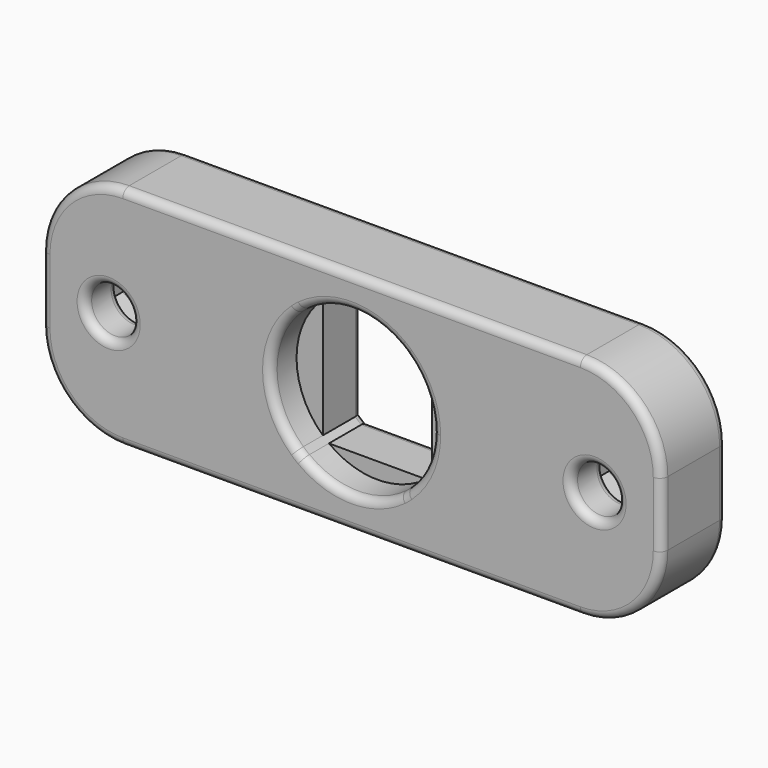
from build123d import *
from build123d import SkipClean  # not in build123d's __all__

# Parameters (mm, degrees)
F0_R     = 1.45
F1_DEPTH = 5
F2_R     = 1.45
F3_DEPTH = 2.5
F5_DEPTH = 2
F6_DEPTH = 5.001
F7_R     = 0.5


with BuildPart() as f1:
    # F0 (on Front) → F1 (new body)
    with BuildSketch(Plane.XZ):
        with BuildLine():
            ThreePointArc((19.125, 2), (17.6605339059, 5.5355339059), (14.125, 7))
            Line((14.125, 7), (-14.125, 7))
            ThreePointArc((-14.125, 7), (-17.6605339059, 5.5355339059), (-19.125, 2))
            Line((-19.125, 2), (-19.125, -2))
            ThreePointArc((-19.125, -2), (-17.6605339059, -5.5355339059), (-14.125, -7))
            Line((-14.125, -7), (14.125, -7))
            ThreePointArc((14.125, -7), (17.6605339059, -5.5355339059), (19.125, -2))
            Line((19.125, -2), (19.125, 2))
        make_face()
        with Locations((-15, 0)):
            Circle(F0_R, mode=Mode.SUBTRACT)
        with Locations((15, 0)):
            Circle(F0_R, mode=Mode.SUBTRACT)
    extrude(amount=-F1_DEPTH)

    # F2 (on face) → F3 (cut)
    with BuildSketch(Plane(origin=(0, 5, 0), x_dir=(-1, 0, 0), z_dir=(0, 1, 0))):
        Polygon((-12.25, -1.5877132403), (-12.25, 1.5877132403), (-15, 3.1754264805), (-17.75, 1.5877132403), (-17.75, -1.5877132403), (-15, -3.1754264805), align=None)
        with Locations((-15, 0)):
            Circle(F2_R, mode=Mode.SUBTRACT)
        Polygon((17.75, 1.5877132403), (15, 3.1754264805), (12.25, 1.5877132403), (12.25, -1.5877132403), (15, -3.1754264805), (17.75, -1.5877132403), align=None)
        with Locations((15, 0)):
            Circle(F2_R, mode=Mode.SUBTRACT)
    extrude(amount=-F3_DEPTH, mode=Mode.SUBTRACT)

    # F4 (on Front) → F5 (cut)
    with BuildSketch(Plane.XZ):
        with BuildLine():
            ThreePointArc((3.375, 3.6890886408), (3.1912885671, 3.8491138307), (3, 4))
            Line((3, 4), (-3, 4))
            ThreePointArc((-3, 4), (-3.1912885671, 3.8491138307), (-3.375, 3.6890886408))
            Line((-3.375, 3.6890886408), (-3.375, -3.6890886408))
            ThreePointArc((-3.375, -3.6890886408), (-3.1912885671, -3.8491138307), (-3, -4))
            Line((-3, -4), (3, -4))
            ThreePointArc((3, -4), (3.1912885671, -3.8491138307), (3.375, -3.6890886408))
            Line((3.375, -3.6890886408), (3.375, 3.6890886408))
        make_face()
        with BuildLine():
            Line((-3, 4), (3, 4))
            ThreePointArc((3, 4), (0, 5), (-3, 4))
        make_face()
        with BuildLine():
            ThreePointArc((5, 0), (4.5757513044, 2.0155644371), (3.375, 3.6890886408))
            Line((3.375, 3.6890886408), (3.375, -3.6890886408))
            ThreePointArc((3.375, -3.6890886408), (4.5757513044, -2.0155644371), (5, 0))
        make_face()
        with BuildLine():
            Line((-3.375, -3.6890886408), (-3.375, 3.6890886408))
            ThreePointArc((-3.375, 3.6890886408), (-5, 0), (-3.375, -3.6890886408))
        make_face()
        with BuildLine():
            ThreePointArc((-3, -4), (0, -5), (3, -4))
            Line((3, -4), (-3, -4))
        make_face()
    extrude(amount=-F5_DEPTH, mode=Mode.SUBTRACT)

    # F4 (on Front) → F6 (cut, through all)
    with BuildSketch(Plane.XZ):
        with BuildLine():
            ThreePointArc((3.375, 3.6890886408), (3.1912885671, 3.8491138307), (3, 4))
            Line((3, 4), (-3, 4))
            ThreePointArc((-3, 4), (-3.1912885671, 3.8491138307), (-3.375, 3.6890886408))
            Line((-3.375, 3.6890886408), (-3.375, -3.6890886408))
            ThreePointArc((-3.375, -3.6890886408), (-3.1912885671, -3.8491138307), (-3, -4))
            Line((-3, -4), (3, -4))
            ThreePointArc((3, -4), (3.1912885671, -3.8491138307), (3.375, -3.6890886408))
            Line((3.375, -3.6890886408), (3.375, 3.6890886408))
        make_face()
    with SkipClean():  # cleaning this boolean's faces spoils the solid; the shape is the same uncleaned
        extrude(amount=-F6_DEPTH, mode=Mode.SUBTRACT)

    # F7
    f7_edges = [f1.edges().sort_by_distance(p)[0] for p in [
        (0, 0, 7),
        (0, 5, 7),
        (19.125, 5, 0),
        (17.660534, 5, -5.535534),
        (17.660534, 5, 5.535534),
        (0, 5, -7),
        (-17.660534, 5, -5.535534),
        (-17.660534, 5, 5.535534),
        (-19.125, 5, 0),
        (-17.75, 5, 0),
        (-16.375, 5, -2.38157),
        (-16.375, 5, 2.38157),
        (-13.625, 5, -2.38157),
        (-13.625, 5, 2.38157),
        (-12.25, 5, 0),
        (3.191289, 5, -3.849114),
        (3.375, 5, 0),
        (3.191289, 5, 3.849114),
        (0, 5, 4),
        (-3.191289, 5, 3.849114),
        (-3.375, 5, 0),
        (-3.191289, 5, -3.849114),
        (0, 5, -4),
        (13.625, 5, -2.38157),
        (16.375, 5, -2.38157),
        (12.25, 5, 0),
        (17.75, 5, 0),
        (13.625, 5, 2.38157),
        (16.375, 5, 2.38157),
        (-16.45, 0, 0),
        (-13.55, 1.25, 0),
        (-16.45, 2.5, 0),
        (13.55, 0, 0),
        (16.45, 1.25, 0),
        (13.55, 2.5, 0),
        (19.125, 0, 0),
        (17.660534, 0, -5.535534),
        (17.660534, 0, 5.535534),
        (0, 0, -7),
        (-17.660534, 0, -5.535534),
        (-17.660534, 0, 5.535534),
        (-19.125, 0, 0),
        (0, 0, -5),
        (3.191289, 0, -3.849114),
        (5, 0, 0),
        (3.191289, 0, 3.849114),
        (0, 0, 5),
        (-3.191289, 0, 3.849114),
        (-5, 0, 0),
        (-3.191289, 0, -3.849114),
    ]]
    fillet(f7_edges, radius=F7_R)


solid = f1.part
